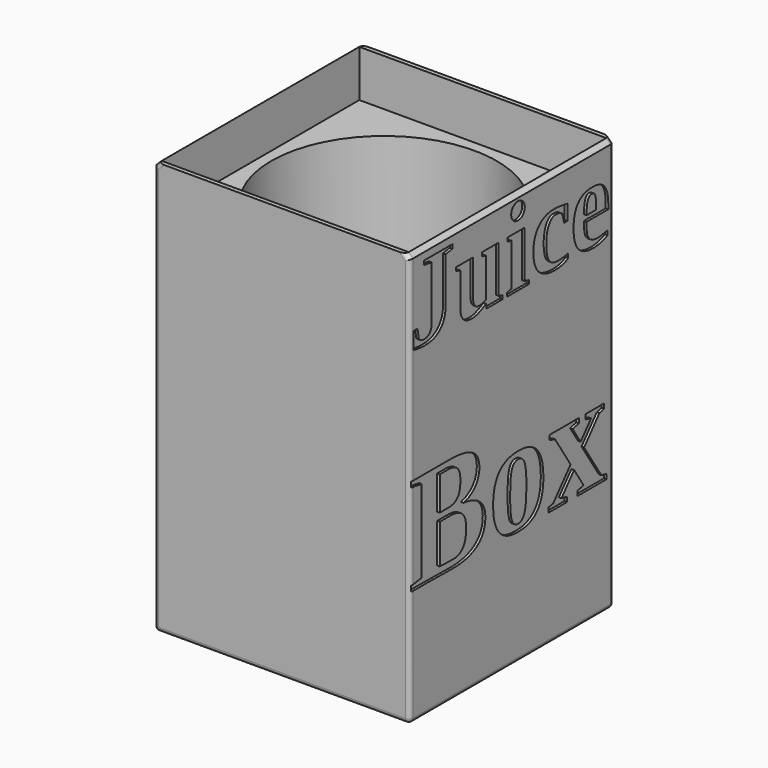
from build123d import *

# Parameters (mm, degrees)
F0_W            = 76.2
F0_H            = 76.2
F1_DEPTH        = 54.61
F2_R            = 33.655
F3_DEPTH        = 106.68
F4_W            = 76.2
F4_H            = 76.2
F4_W_2          = 73.66
F4_H_2          = 73.66
F5_DEPTH        = 13.97
F6_SIZE         = 1.26999
F7_TEXT_SIZE    = 33.7424756106
F7_TEXT_SIZE_2  = 44.1939284096
F9_DEPTH        = 0.762
F8_TEXT_SIZE    = 33.7424756106
F8_TEXT_SIZE_2  = 44.1939284096
F10_DEPTH       = 0.762
F11_TEXT_SIZE   = 17.3304904051
F11_TEXT_SIZE_2 = 28.0873998741
F12_DEPTH       = 0.762
F13_T1_DEPTH    = 8.1460370821
F13_T3_DEPTH    = 123.82501
F13_T5_DEPTH    = 8.1460370821
F13_T7_DEPTH    = 73.66
F13_T9_DEPTH    = 73.66
F13_S13_W       = 1.2954
F13_S13_H       = 1.2954
F13_T14_DEPTH   = 1.2954
F13_S19_W       = 1.2954
F13_S19_H       = 1.2954
F13_T20_DEPTH   = 1.2954
F13_S25_W       = 1.2954
F13_S25_H       = 1.2954
F13_T26_DEPTH   = 1.2954
F13_S31_W       = 1.2954
F13_S31_H       = 1.2954
F13_T32_DEPTH   = 1.2954


# Not quite as in the source:
# - a fillet or chamfer that OpenCascade refuses, or shapes differently, is made with other operations: its cross-section is extruded or revolved along the edge and cut away or added
# - a fillet or chamfer is up to 0.001 mm smaller than in the source, because OpenCascade refuses the exact size
# - Text() gives the source's letters only with a copy of the font that has no kerning and outlines rounded to 1/6400 em; it was checked with that copy


with BuildPart() as f1:
    # F0 (on Top) → F1 (new body, symmetric)
    with BuildSketch(Plane.XY):
        Rectangle(F0_W, F0_H)
    extrude(amount=F1_DEPTH, both=True)

    # F2 (on face) → F3 (cut)
    with BuildSketch(Plane.XY.offset(54.61)):
        Circle(F2_R)
    extrude(amount=-F3_DEPTH, mode=Mode.SUBTRACT)

    # F4 (on face) → F5 (join)
    with BuildSketch(Plane.XY.offset(54.61)):
        Rectangle(F4_W, F4_H)
        Rectangle(F4_W_2, F4_H_2, mode=Mode.SUBTRACT)
    extrude(amount=F5_DEPTH)

    # F6 (size 1.27 in the source; OpenCascade refuses exactly that, so slightly less here)
    f6_edges = [f1.edges().sort_by_distance(p)[0] for p in [
        (-38.1, 0, 68.58),
        (38.1, 0, 68.58),
    ]]
    chamfer(f6_edges, length=F6_SIZE)

    # F7 (on face) → F9 (cut)
    with BuildSketch(Plane(origin=(-38.1, 0, 0), x_dir=(0, -1, 0), z_dir=(-1, 0, 0))):
        with Locations((-38.1, 42.8985477543)):
            Text('Juice', F7_TEXT_SIZE, font='Tinos', font_style=FontStyle.BOLD, text_align=(TextAlign.LEFT, TextAlign.BOTTOM))
        with Locations((-38.1, -19.6095953063)):
            Text('Box', F7_TEXT_SIZE_2, font='Tinos', font_style=FontStyle.BOLD, text_align=(TextAlign.LEFT, TextAlign.BOTTOM))
    extrude(amount=-F9_DEPTH, mode=Mode.SUBTRACT)

    # F8 (on face) → F10 (cut)
    with BuildSketch(Plane.YZ.offset(38.1)):
        with Locations((-38.1, 43.0154175604)):
            Text('Juice', F8_TEXT_SIZE, font='Tinos', font_style=FontStyle.BOLD, text_align=(TextAlign.LEFT, TextAlign.BOTTOM))
        with Locations((-38.1, -19.9795836881)):
            Text('Box', F8_TEXT_SIZE_2, font='Tinos', font_style=FontStyle.BOLD, text_align=(TextAlign.LEFT, TextAlign.BOTTOM))
    extrude(amount=-F10_DEPTH, mode=Mode.SUBTRACT)

    # F11 (on face) → F12 (cut)
    with BuildSketch(Plane(origin=(0, 0, -54.61), x_dir=(1, 0, 0), z_dir=(0, 0, -1))):
        with Locations((-31.75, 15.336368498)):
            Text('Michelle', F11_TEXT_SIZE, font='Tinos', font_style=FontStyle.BOLDITALIC, text_align=(TextAlign.LEFT, TextAlign.BOTTOM))
        with Locations((-30.0788152963, -25.5634319037)):
            Text('Kelly', F11_TEXT_SIZE_2, font='Tinos', font_style=FontStyle.BOLDITALIC, text_align=(TextAlign.LEFT, TextAlign.BOTTOM))
    extrude(amount=-F12_DEPTH, mode=Mode.SUBTRACT)

    # F13: fillet of radius 1.27 on 12 edges, made by hand

    # F13_s2 → F13_t1 (cut)
    with BuildSketch(Plane(origin=(-12.3599409697, 0, 12.3599409697), x_dir=(0, 1, 0), z_dir=(-0.7071067812, 0, 0.7071067812))):
        with BuildLine():
            ThreePointArc((38.1, -73.2661328759), (37.7280256121, -74.164158488), (36.83, -74.5361328759))
            Line((36.83, -74.5361328759), (38.1, -74.5361328759))
            Line((38.1, -74.5361328759), (38.1, -73.2661328759))
        make_face()
        with BuildLine():
            ThreePointArc((-36.83, -74.5361328759), (-37.7280256121, -74.164158488), (-38.1, -73.2661328759))
            Line((-38.1, -73.2661328759), (-38.1, -74.5361328759))
            Line((-38.1, -74.5361328759), (-36.83, -74.5361328759))
        make_face()
    extrude(amount=F13_T1_DEPTH, mode=Mode.SUBTRACT)

    # F13_s4 → F13_t3 (cut)
    with BuildSketch(Plane.XY.offset(-53.34)):
        with BuildLine():
            ThreePointArc((36.83, 38.1), (37.7280256121, 37.7280256121), (38.1, 36.83))
            Line((38.1, 36.83), (38.1, 38.1))
            Line((38.1, 38.1), (36.83, 38.1))
        make_face()
        with BuildLine():
            ThreePointArc((-36.83, 38.1), (-37.7280256121, 37.7280256121), (-38.1, 36.83))
            Line((-38.1, 36.83), (-38.1, 38.1))
            Line((-38.1, 38.1), (-36.83, 38.1))
        make_face()
        with BuildLine():
            ThreePointArc((-38.1, -36.83), (-37.7280256121, -37.7280256121), (-36.83, -38.1))
            Line((-36.83, -38.1), (-38.1, -38.1))
            Line((-38.1, -38.1), (-38.1, -36.83))
        make_face()
        with BuildLine():
            ThreePointArc((38.1, -36.83), (37.7280256121, -37.7280256121), (36.83, -38.1))
            Line((36.83, -38.1), (38.1, -38.1))
            Line((38.1, -38.1), (38.1, -36.83))
        make_face()
    extrude(amount=F13_T3_DEPTH, mode=Mode.SUBTRACT)

    # F13_s6 → F13_t5 (cut)
    with BuildSketch(Plane(origin=(18.1200590303, 0, 18.1200590303), x_dir=(0, 1, 0), z_dir=(-0.7071067812, 0, -0.7071067812))):
        with BuildLine():
            ThreePointArc((38.1, -73.2661328759), (37.7280256121, -74.164158488), (36.83, -74.5361328759))
            Line((36.83, -74.5361328759), (38.1, -74.5361328759))
            Line((38.1, -74.5361328759), (38.1, -73.2661328759))
        make_face()
        with BuildLine():
            ThreePointArc((-36.83, -74.5361328759), (-37.7280256121, -74.164158488), (-38.1, -73.2661328759))
            Line((-38.1, -73.2661328759), (-38.1, -74.5361328759))
            Line((-38.1, -74.5361328759), (-36.83, -74.5361328759))
        make_face()
    extrude(amount=F13_T5_DEPTH, mode=Mode.SUBTRACT)

    # F13_s8 → F13_t7 (cut)
    with BuildSketch(Plane.YZ.offset(-36.83)):
        with BuildLine():
            ThreePointArc((-36.83, -54.61), (-37.7280256121, -54.2380256121), (-38.1, -53.34))
            Line((-38.1, -53.34), (-38.1, -54.61))
            Line((-38.1, -54.61), (-36.83, -54.61))
        make_face()
        with BuildLine():
            ThreePointArc((38.1, -53.34), (37.7280256121, -54.2380256121), (36.83, -54.61))
            Line((36.83, -54.61), (38.1, -54.61))
            Line((38.1, -54.61), (38.1, -53.34))
        make_face()
    extrude(amount=F13_T7_DEPTH, mode=Mode.SUBTRACT)

    # F13_s10 → F13_t9 (cut)
    with BuildSketch(Plane.XZ.offset(-36.83)):
        with BuildLine():
            ThreePointArc((-38.1, -53.34), (-37.7280256121, -54.2380256121), (-36.83, -54.61))
            Line((-36.83, -54.61), (-38.1, -54.61))
            Line((-38.1, -54.61), (-38.1, -53.34))
        make_face()
        with BuildLine():
            ThreePointArc((36.83, -54.61), (37.7280256121, -54.2380256121), (38.1, -53.34))
            Line((38.1, -53.34), (38.1, -54.61))
            Line((38.1, -54.61), (36.83, -54.61))
        make_face()
    extrude(amount=F13_T9_DEPTH, mode=Mode.SUBTRACT)


with BuildPart() as f13_tool12:
    # F13_s13 → F13_t14 (new body)
    with BuildSketch(Plane.XZ.offset(-36.83)):
        with Locations((37.4777, -53.9877)):
            Rectangle(F13_S13_W, F13_S13_H)
    extrude(amount=-F13_T14_DEPTH)

    # F13_s15 → F13_t16 (revolve, cut)
    with BuildSketch(Plane(origin=(36.83, 36.83, -53.34), x_dir=(-0.7071067812, 0, 0.7071067812), z_dir=(-0.7071067812, 0, -0.7071067812))):
        with BuildLine():
            ThreePointArc((0, -1.27), (1.27, 0), (0, 1.27))
            Line((0, 1.27), (0, -1.27))
        make_face()
    revolve(axis=Axis((36.83, 36.83, -53.34), (0, 1, 0)), mode=Mode.SUBTRACT)


with BuildPart() as f1_1:
    add(f1.part)

    # F13_t11: cut F13_tool12
    add(f13_tool12.part, mode=Mode.SUBTRACT)


with BuildPart() as f13_tool18:
    # F13_s19 → F13_t20 (new body)
    with BuildSketch(Plane.XZ.offset(-36.83)):
        with Locations((-37.4777, -53.9877)):
            Rectangle(F13_S19_W, F13_S19_H)
    extrude(amount=-F13_T20_DEPTH)

    # F13_s21 → F13_t22 (revolve, cut)
    with BuildSketch(Plane(origin=(-36.83, 36.83, -53.34), x_dir=(0.7071067812, 0, 0.7071067812), z_dir=(-0.7071067812, 0, 0.7071067812))):
        with BuildLine():
            ThreePointArc((0, -1.27), (1.27, 0), (0, 1.27))
            Line((0, 1.27), (0, -1.27))
        make_face()
    revolve(axis=Axis((-36.83, 36.83, -53.34), (0, 1, 0)), mode=Mode.SUBTRACT)


with BuildPart() as f1_2:
    add(f1_1.part)

    # F13_t17: cut F13_tool18
    add(f13_tool18.part, mode=Mode.SUBTRACT)


with BuildPart() as f13_tool24:
    # F13_s25 → F13_t26 (new body)
    with BuildSketch(Plane.YZ.offset(-36.83)):
        with Locations((-37.4777, -53.9877)):
            Rectangle(F13_S25_W, F13_S25_H)
    extrude(amount=-F13_T26_DEPTH)

    # F13_s27 → F13_t28 (revolve, cut)
    with BuildSketch(Plane(origin=(-36.83, -36.83, -53.34), x_dir=(0, 0.7071067812, 0.7071067812), z_dir=(0, -0.7071067812, 0.7071067812))):
        with BuildLine():
            ThreePointArc((0, -1.27), (1.27, 0), (0, 1.27))
            Line((0, 1.27), (0, -1.27))
        make_face()
    revolve(axis=Axis((-36.83, -36.83, -53.34), (-1, 0, 0)), mode=Mode.SUBTRACT)


with BuildPart() as f1_3:
    add(f1_2.part)

    # F13_t23: cut F13_tool24
    add(f13_tool24.part, mode=Mode.SUBTRACT)


with BuildPart() as f13_tool30:
    # F13_s31 → F13_t32 (new body)
    with BuildSketch(Plane.XY.offset(-53.34)):
        with Locations((37.4777, -37.4777)):
            Rectangle(F13_S31_W, F13_S31_H)
    extrude(amount=-F13_T32_DEPTH)

    # F13_s33 → F13_t34 (revolve, cut)
    with BuildSketch(Plane(origin=(36.83, -36.83, -53.34), x_dir=(-0.7071067812, 0.7071067812, 0), z_dir=(-0.7071067812, -0.7071067812, 0))):
        with BuildLine():
            ThreePointArc((0, -1.27), (1.27, 0), (0, 1.27))
            Line((0, 1.27), (0, -1.27))
        make_face()
    revolve(axis=Axis((36.83, -36.83, -53.34), (0, 0, -1)), mode=Mode.SUBTRACT)


with BuildPart() as f1_4:
    add(f1_3.part)

    # F13_t29: cut F13_tool30
    add(f13_tool30.part, mode=Mode.SUBTRACT)


solid = f1_4.part
